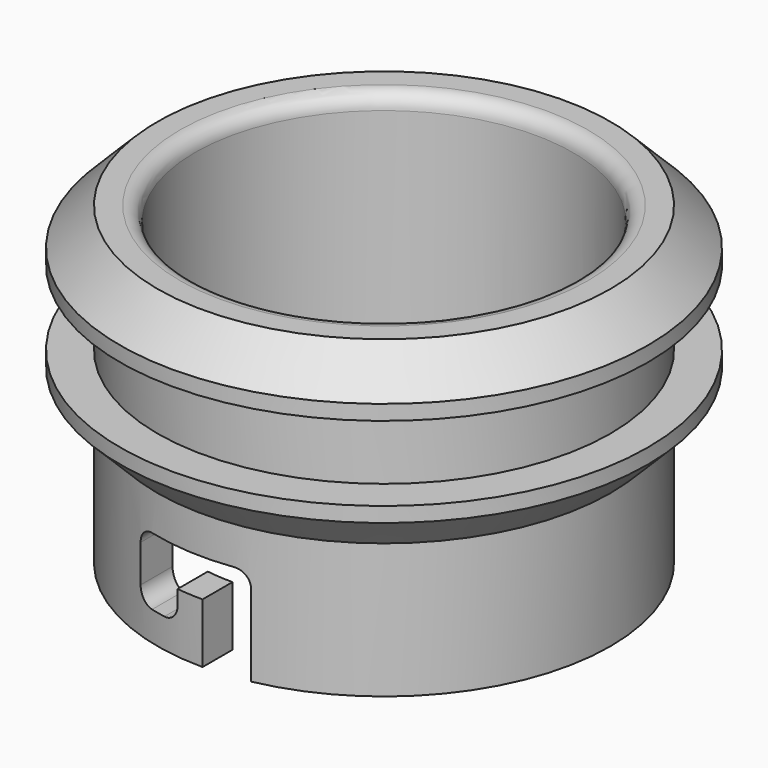
from build123d import *

# Parameters (mm, degrees)
F0_R      = 30.25
F0_R_2    = 25.25
F1_DEPTH  = 18
F2_R      = 35.25
F2_R_2    = 30.25
F2_R_3    = 25.25
F3_DEPTH  = 7
F4_R      = 30.25
F4_R_2    = 25.25
F5_DEPTH  = 10
F6_R      = 35.25
F6_R_2    = 30.25
F6_R_3    = 25.25
F7_DEPTH  = 7
F8_R      = 2
F10_DEPTH = 50
F11_R     = 2
F13_DEPTH = 50
F14_R     = 2
F15_SIZE2 = 4.99999
F15_SIZE  = 4.99999


# Not quite as in the source:
# - a fillet or chamfer is up to 0.001 mm smaller than in the source, because OpenCascade refuses the exact size


with BuildPart() as f1:
    # F0 (on Top) → F1 (new body)
    with BuildSketch(Plane.XY):
        Circle(F0_R)
        Circle(F0_R_2, mode=Mode.SUBTRACT)
    extrude(amount=F1_DEPTH)

    # F2 (on face) → F3 (join)
    with BuildSketch(Plane.XY.offset(18)):
        Circle(F2_R)
        Circle(F2_R_2, mode=Mode.SUBTRACT)
        Circle(F2_R_2)
        Circle(F2_R_3, mode=Mode.SUBTRACT)
    extrude(amount=F3_DEPTH)

    # F4 (on face) → F5 (join)
    with BuildSketch(Plane.XY.offset(25)):
        Circle(F4_R)
        Circle(F4_R_2, mode=Mode.SUBTRACT)
    extrude(amount=F5_DEPTH)

    # F6 (on face) → F7 (join)
    with BuildSketch(Plane.XY.offset(35)):
        Circle(F6_R)
        Circle(F6_R_2, mode=Mode.SUBTRACT)
        Circle(F6_R_2)
        Circle(F6_R_3, mode=Mode.SUBTRACT)
    extrude(amount=F7_DEPTH)

    # F8
    f8_edges = [f1.edges().sort_by_distance(p)[0] for p in [
        (-25.25, 0, 42),
    ]]
    fillet(f8_edges, radius=F8_R)

    # F9 (on Front) → F10 (cut)
    with BuildSketch(Plane.XZ):
        Polygon((-6, 0), (0, 0), (0, 8.0120034479), (3.5, 8.0120034479), (3.5, 4), (9.5, 4), (9.5, 13), (-6, 13), align=None)
    extrude(amount=-F10_DEPTH, mode=Mode.SUBTRACT)

    # F11
    f11_edges = [f1.edges().sort_by_distance(p)[0] for p in [
        (9.5, 26.05713, 13),
        (-6, 27.08788, 13),
        (3.5, 27.526544, 4),
        (9.5, 26.05713, 4),
    ]]
    fillet(f11_edges, radius=F11_R)

    # F12 (on Front) → F13 (cut)
    with BuildSketch(Plane.XZ):
        Polygon((-0.0314122736, -0.0527559742), (5.9685877264, -0.0527559742), (5.9685877264, 12.9472440258), (-9.5314122736, 12.9472440258), (-9.5314122736, 3.9472440258), (-3.5314122736, 3.9472440258), (-3.5314122736, 7.9592474737), (-0.0314122736, 7.9592474737), align=None)
    extrude(amount=F13_DEPTH, mode=Mode.SUBTRACT)

    # F14
    f14_edges = [f1.edges().sort_by_distance(p)[0] for p in [
        (-9.531412, -26.045535, 12.947244),
        (-9.531412, -26.045535, 3.947244),
        (-3.531412, -27.522498, 3.947244),
        (5.968588, -27.094881, 12.947244),
    ]]
    fillet(f14_edges, radius=F14_R)

    # F15 (size 5 and 5 in the source; OpenCascade refuses exactly that, so slightly less here)
    f15_edges = [f1.edges().sort_by_distance(p)[0] for p in [
        (-35.25, 0, 18),
        (-35.25, 0, 42),
    ]]
    chamfer(f15_edges, length=F15_SIZE, length2=F15_SIZE2)


solid = f1.part
